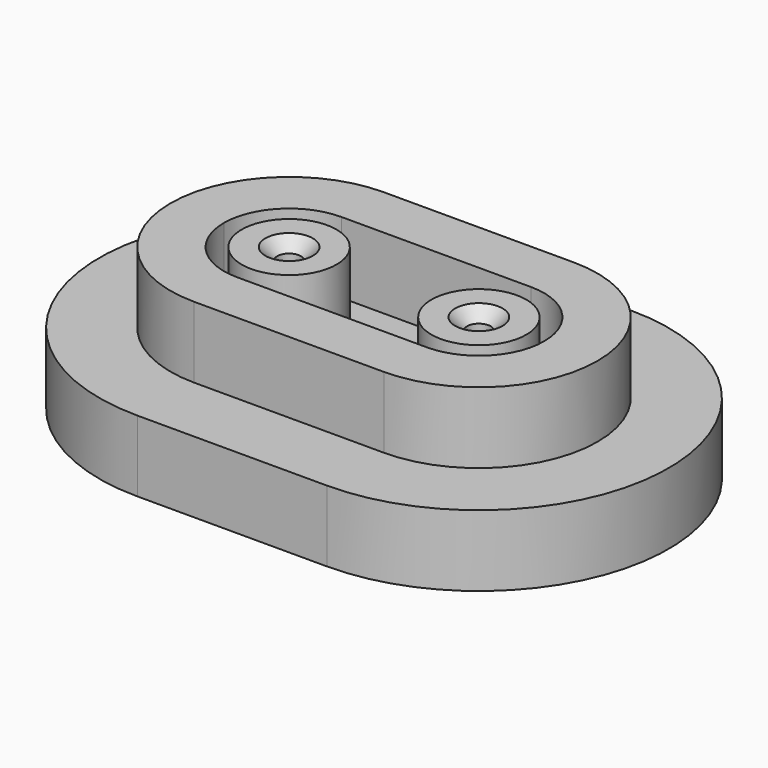
from build123d import *

# Parameters (mm, degrees)
F0_R     = 50.8
F0_R_2   = 25.4
F0_R_3   = 12.7
F1_DEPTH = 76.2
F2_START = -76.2
F2_DEPTH = 76.2
F3_START = -127
F3_DEPTH = 25.4
F4_DEPTH = 76.2


# Not quite as in the source:
# - a pattern or mirror of a feature is missing from the dataset's text; its kind, count and spacing are read off the source's solid


with BuildPart() as f1:
    # F0 (on Top) → F1 (new body)
    with BuildSketch(Plane.XY):
        with BuildLine():
            Line((-101.6, -127), (101.6, -127))
            ThreePointArc((101.6, -127), (191.4025612107, -89.8025612107), (228.6, 0))
            ThreePointArc((228.6, 0), (191.4025612107, 89.8025612107), (101.6, 127))
            Line((101.6, 127), (-101.6, 127))
            ThreePointArc((-101.6, 127), (-191.4025612107, 89.8025612107), (-228.6, 0))
            ThreePointArc((-228.6, 0), (-191.4025612107, -89.8025612107), (-101.6, -127))
        make_face()
        with BuildLine():
            ThreePointArc((203.2, 0), (173.4420489686, -71.8420489686), (101.6, -101.6))
            Line((101.6, -101.6), (-101.6, -101.6))
            ThreePointArc((-101.6, -101.6), (-173.4420489686, -71.8420489686), (-203.2, 0))
            ThreePointArc((-203.2, 0), (-173.4420489686, 71.8420489686), (-101.6, 101.6))
            Line((-101.6, 101.6), (101.6, 101.6))
            ThreePointArc((101.6, 101.6), (173.4420489686, 71.8420489686), (203.2, 0))
        make_face(mode=Mode.SUBTRACT)
        with BuildLine():
            Line((-101.6, -101.6), (101.6, -101.6))
            ThreePointArc((101.6, -101.6), (173.4420489686, -71.8420489686), (203.2, 0))
            ThreePointArc((203.2, 0), (173.4420489686, 71.8420489686), (101.6, 101.6))
            Line((101.6, 101.6), (-101.6, 101.6))
            ThreePointArc((-101.6, 101.6), (-173.4420489686, 71.8420489686), (-203.2, 0))
            ThreePointArc((-203.2, 0), (-173.4420489686, -71.8420489686), (-101.6, -101.6))
        make_face()
        with BuildLine():
            Line((-101.6, 69.85), (101.6, 69.85))
            ThreePointArc((101.6, 69.85), (150.9914086659, 49.3914086659), (171.45, 0))
            ThreePointArc((171.45, 0), (150.9914086659, -49.3914086659), (101.6, -69.85))
            Line((101.6, -69.85), (-101.6, -69.85))
            ThreePointArc((-101.6, -69.85), (-150.9914086659, -49.3914086659), (-171.45, 0))
            ThreePointArc((-171.45, 0), (-150.9914086659, 49.3914086659), (-101.6, 69.85))
        make_face(mode=Mode.SUBTRACT)
        with BuildLine():
            ThreePointArc((171.45, 0), (150.9914086659, 49.3914086659), (101.6, 69.85))
            Line((101.6, 69.85), (-101.6, 69.85))
            ThreePointArc((-101.6, 69.85), (-150.9914086659, 49.3914086659), (-171.45, 0))
            ThreePointArc((-171.45, 0), (-150.9914086659, -49.3914086659), (-101.6, -69.85))
            Line((-101.6, -69.85), (101.6, -69.85))
            ThreePointArc((101.6, -69.85), (150.9914086659, -49.3914086659), (171.45, 0))
        make_face()
        with Locations((-101.6, 0)):
            Circle(F0_R, mode=Mode.SUBTRACT)
        with Locations((101.6, 0)):
            Circle(F0_R, mode=Mode.SUBTRACT)
        with Locations((-101.6, 0)):
            Circle(F0_R)
        with Locations((-101.6, 0)):
            Circle(F0_R_2, mode=Mode.SUBTRACT)
        with Locations((101.6, 0)):
            Circle(F0_R)
        with Locations((101.6, 0)):
            Circle(F0_R_2, mode=Mode.SUBTRACT)
        with Locations((-101.6, 0)):
            Circle(F0_R_2)
        with Locations((-101.6, 0)):
            Circle(F0_R_3, mode=Mode.SUBTRACT)
        with Locations((101.6, 0)):
            Circle(F0_R_2)
        with Locations((101.6, 0)):
            Circle(F0_R_3, mode=Mode.SUBTRACT)
    extrude(amount=-F1_DEPTH)

    # F0 (on Top) → F2 (join)
    with BuildSketch(Plane.XY.offset(F2_START)):
        with BuildLine():
            Line((-101.6, -203.2), (101.6, -203.2))
            ThreePointArc((101.6, -203.2), (245.2840979371, -143.6840979371), (304.8, 0))
            ThreePointArc((304.8, 0), (245.2840979371, 143.6840979371), (101.6, 203.2))
            Line((101.6, 203.2), (-101.6, 203.2))
            ThreePointArc((-101.6, 203.2), (-245.2840979371, 143.6840979371), (-304.8, 0))
            ThreePointArc((-304.8, 0), (-245.2840979371, -143.6840979371), (-101.6, -203.2))
        make_face()
        with BuildLine():
            ThreePointArc((228.6, 0), (191.4025612107, -89.8025612107), (101.6, -127))
            Line((101.6, -127), (-101.6, -127))
            ThreePointArc((-101.6, -127), (-191.4025612107, -89.8025612107), (-228.6, 0))
            ThreePointArc((-228.6, 0), (-191.4025612107, 89.8025612107), (-101.6, 127))
            Line((-101.6, 127), (101.6, 127))
            ThreePointArc((101.6, 127), (191.4025612107, 89.8025612107), (228.6, 0))
        make_face(mode=Mode.SUBTRACT)
        with BuildLine():
            Line((-101.6, -127), (101.6, -127))
            ThreePointArc((101.6, -127), (191.4025612107, -89.8025612107), (228.6, 0))
            ThreePointArc((228.6, 0), (191.4025612107, 89.8025612107), (101.6, 127))
            Line((101.6, 127), (-101.6, 127))
            ThreePointArc((-101.6, 127), (-191.4025612107, 89.8025612107), (-228.6, 0))
            ThreePointArc((-228.6, 0), (-191.4025612107, -89.8025612107), (-101.6, -127))
        make_face()
        with BuildLine():
            ThreePointArc((203.2, 0), (173.4420489686, -71.8420489686), (101.6, -101.6))
            Line((101.6, -101.6), (-101.6, -101.6))
            ThreePointArc((-101.6, -101.6), (-173.4420489686, -71.8420489686), (-203.2, 0))
            ThreePointArc((-203.2, 0), (-173.4420489686, 71.8420489686), (-101.6, 101.6))
            Line((-101.6, 101.6), (101.6, 101.6))
            ThreePointArc((101.6, 101.6), (173.4420489686, 71.8420489686), (203.2, 0))
        make_face(mode=Mode.SUBTRACT)
        with BuildLine():
            Line((-101.6, -101.6), (101.6, -101.6))
            ThreePointArc((101.6, -101.6), (173.4420489686, -71.8420489686), (203.2, 0))
            ThreePointArc((203.2, 0), (173.4420489686, 71.8420489686), (101.6, 101.6))
            Line((101.6, 101.6), (-101.6, 101.6))
            ThreePointArc((-101.6, 101.6), (-173.4420489686, 71.8420489686), (-203.2, 0))
            ThreePointArc((-203.2, 0), (-173.4420489686, -71.8420489686), (-101.6, -101.6))
        make_face()
        with BuildLine():
            Line((-101.6, 69.85), (101.6, 69.85))
            ThreePointArc((101.6, 69.85), (150.9914086659, 49.3914086659), (171.45, 0))
            ThreePointArc((171.45, 0), (150.9914086659, -49.3914086659), (101.6, -69.85))
            Line((101.6, -69.85), (-101.6, -69.85))
            ThreePointArc((-101.6, -69.85), (-150.9914086659, -49.3914086659), (-171.45, 0))
            ThreePointArc((-171.45, 0), (-150.9914086659, 49.3914086659), (-101.6, 69.85))
        make_face(mode=Mode.SUBTRACT)
        with BuildLine():
            ThreePointArc((171.45, 0), (150.9914086659, 49.3914086659), (101.6, 69.85))
            Line((101.6, 69.85), (-101.6, 69.85))
            ThreePointArc((-101.6, 69.85), (-150.9914086659, 49.3914086659), (-171.45, 0))
            ThreePointArc((-171.45, 0), (-150.9914086659, -49.3914086659), (-101.6, -69.85))
            Line((-101.6, -69.85), (101.6, -69.85))
            ThreePointArc((101.6, -69.85), (150.9914086659, -49.3914086659), (171.45, 0))
        make_face()
        with Locations((-101.6, 0)):
            Circle(F0_R, mode=Mode.SUBTRACT)
        with Locations((101.6, 0)):
            Circle(F0_R, mode=Mode.SUBTRACT)
        with Locations((-101.6, 0)):
            Circle(F0_R)
        with Locations((-101.6, 0)):
            Circle(F0_R_2, mode=Mode.SUBTRACT)
        with Locations((-101.6, 0)):
            Circle(F0_R_2)
        with Locations((-101.6, 0)):
            Circle(F0_R_3, mode=Mode.SUBTRACT)
        with Locations((101.6, 0)):
            Circle(F0_R)
        with Locations((101.6, 0)):
            Circle(F0_R_2, mode=Mode.SUBTRACT)
        with Locations((101.6, 0)):
            Circle(F0_R_2)
        with Locations((101.6, 0)):
            Circle(F0_R_3, mode=Mode.SUBTRACT)
    extrude(amount=-F2_DEPTH)

    # F0 (on Top) → F3 (cut)
    with BuildSketch(Plane.XY.offset(F3_START)):
        with BuildLine():
            Line((-101.6, -101.6), (101.6, -101.6))
            ThreePointArc((101.6, -101.6), (173.4420489686, -71.8420489686), (203.2, 0))
            ThreePointArc((203.2, 0), (173.4420489686, 71.8420489686), (101.6, 101.6))
            Line((101.6, 101.6), (-101.6, 101.6))
            ThreePointArc((-101.6, 101.6), (-173.4420489686, 71.8420489686), (-203.2, 0))
            ThreePointArc((-203.2, 0), (-173.4420489686, -71.8420489686), (-101.6, -101.6))
        make_face()
        with BuildLine():
            Line((-101.6, 69.85), (101.6, 69.85))
            ThreePointArc((101.6, 69.85), (150.9914086659, 49.3914086659), (171.45, 0))
            ThreePointArc((171.45, 0), (150.9914086659, -49.3914086659), (101.6, -69.85))
            Line((101.6, -69.85), (-101.6, -69.85))
            ThreePointArc((-101.6, -69.85), (-150.9914086659, -49.3914086659), (-171.45, 0))
            ThreePointArc((-171.45, 0), (-150.9914086659, 49.3914086659), (-101.6, 69.85))
        make_face(mode=Mode.SUBTRACT)
        with BuildLine():
            ThreePointArc((171.45, 0), (150.9914086659, 49.3914086659), (101.6, 69.85))
            Line((101.6, 69.85), (-101.6, 69.85))
            ThreePointArc((-101.6, 69.85), (-150.9914086659, 49.3914086659), (-171.45, 0))
            ThreePointArc((-171.45, 0), (-150.9914086659, -49.3914086659), (-101.6, -69.85))
            Line((-101.6, -69.85), (101.6, -69.85))
            ThreePointArc((101.6, -69.85), (150.9914086659, -49.3914086659), (171.45, 0))
        make_face()
        with Locations((-101.6, 0)):
            Circle(F0_R, mode=Mode.SUBTRACT)
        with Locations((101.6, 0)):
            Circle(F0_R, mode=Mode.SUBTRACT)
        with Locations((101.6, 0)):
            Circle(F0_R)
        with Locations((101.6, 0)):
            Circle(F0_R_2, mode=Mode.SUBTRACT)
        with Locations((101.6, 0)):
            Circle(F0_R_2)
        with Locations((101.6, 0)):
            Circle(F0_R_3, mode=Mode.SUBTRACT)
        with Locations((-101.6, 0)):
            Circle(F0_R)
        with Locations((-101.6, 0)):
            Circle(F0_R_2, mode=Mode.SUBTRACT)
        with Locations((-101.6, 0)):
            Circle(F0_R_2)
        with Locations((-101.6, 0)):
            Circle(F0_R_3, mode=Mode.SUBTRACT)
        with Locations((-101.6, 0)):
            Circle(F0_R_3)
        with Locations((101.6, 0)):
            Circle(F0_R_3)
    extrude(amount=-F3_DEPTH, mode=Mode.SUBTRACT)

    # F0 (on Top) → F4 (cut)
    with BuildSketch(Plane.XY):
        with BuildLine():
            ThreePointArc((171.45, 0), (150.9914086659, 49.3914086659), (101.6, 69.85))
            Line((101.6, 69.85), (-101.6, 69.85))
            ThreePointArc((-101.6, 69.85), (-150.9914086659, 49.3914086659), (-171.45, 0))
            ThreePointArc((-171.45, 0), (-150.9914086659, -49.3914086659), (-101.6, -69.85))
            Line((-101.6, -69.85), (101.6, -69.85))
            ThreePointArc((101.6, -69.85), (150.9914086659, -49.3914086659), (171.45, 0))
        make_face()
        with Locations((-101.6, 0)):
            Circle(F0_R, mode=Mode.SUBTRACT)
        with Locations((101.6, 0)):
            Circle(F0_R, mode=Mode.SUBTRACT)
    extrude(amount=-F4_DEPTH, mode=Mode.SUBTRACT)

    # F5 (on Front) → F6 (revolve, cut)
    with BuildSketch(Plane.XZ):
        Polygon((127, 0), (101.6, 0), (101.6, -12.7), (114.3, -12.7), align=None)
    f6 = revolve(axis=Axis((101.6, 0, -6.35), (0, 0, -1)), mode=Mode.SUBTRACT)

    # F6_copies: F6 across plane
    add(f6.mirror(Plane(origin=(0, 0, 0), x_dir=(0, 0, -1), z_dir=(-1, 0, 0))), mode=Mode.SUBTRACT)


solid = f1.part
